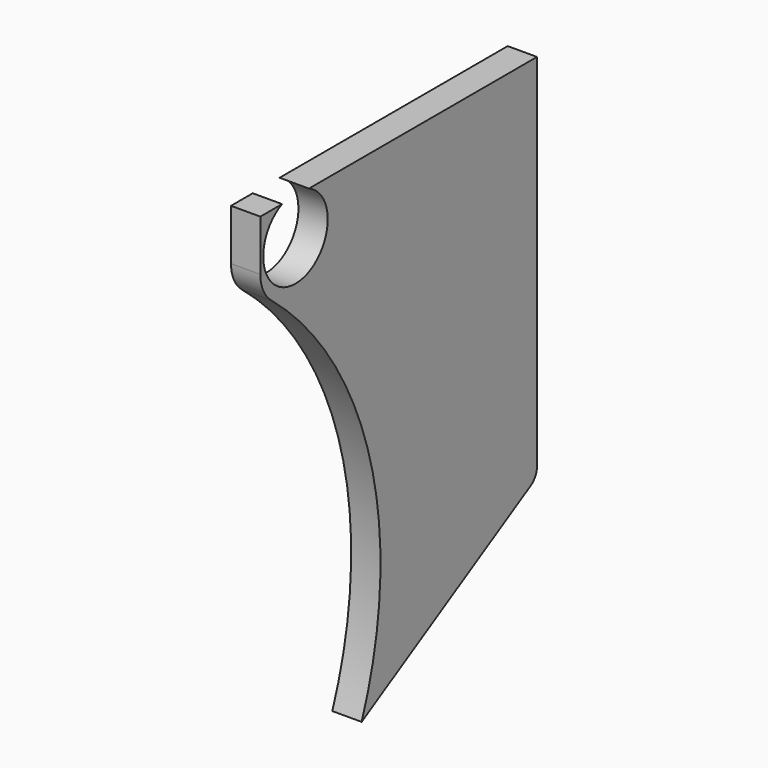
from build123d import *

# Parameters (mm, degrees)
F1_DEPTH     = 34
F2_R         = 5
F3_T         = -2.4
F5_DEPTH     = 31.6
F6_R         = 2.5
F7_DEPTH     = 34.001
F8_R         = 5
F9_T         = 2.4
F9_T3_DEPTH  = 10.7666522226
F9_T5_DEPTH  = 36.6379168457
F9_T7_DEPTH  = 39.0950180144
F9_T9_DEPTH  = 53.9897706946
F9_T11_DEPTH = 38.5655287546
F9_T13_DEPTH = 38.5655287546
F9_T15_DEPTH = 34
F9_T17_DEPTH = 38.8
F9_T20_ANGLE = 72.0602715047
F9_T22_ANGLE = 0.4928779222
F9_T24_ANGLE = 94.6188464687
F9_T26_ANGLE = 72.0602715047
F9_T28_ANGLE = 0.4928779222
F9_T30_ANGLE = 94.6188464687
F9_T32_ANGLE = 60.000000001
F9_T34_ANGLE = 60.000000001
F11_R        = 2.5
F12_DEPTH    = 4
F13_R        = 5
F13_R_2      = 2.5
F14_DEPTH    = 31.6
F15_W        = 10
F15_H        = 5
F16_DEPTH    = 34
F17_R        = 2.1082
F18_DEPTH    = 95.001
F19_W        = 189.8932904005
F19_H        = 164.366655983
F21_DEPTH    = 9.401
F23_DEPTH    = 25
F24_W        = 160.8902737498
F24_H        = 109.9677272141
F25_DEPTH    = 20.601
F20_R        = 5.5
F26_DEPTH    = 4.001
F28_DEPTH    = 4.001


# Not quite as in the source:
# - a shell that OpenCascade refuses in one call is made with other operations: the cavity is built on its own and cut out


with BuildPart() as f1:
    # F0 (on Right) → F1 (new body)
    with BuildSketch(Plane.YZ):
        with BuildLine():
            Line((28.1775091127, -64.6757430287), (50, -52.0765220406))
            Line((50, -52.0765220406), (50, 0))
            Line((50, 0), (0, 0))
            Line((0, 0), (0, -9.3767308061))
            ThreePointArc((0, -9.3767308061), (-15.3280037593, -98.3216569078), (-77.5220977637, -32.9149122293))
            Line((-77.5220977637, -32.9149122293), (-87.5160827584, -32.9149122293))
            ThreePointArc((-87.5160827584, -32.9149122293), (-82.2268855449, -79.5356128475), (-45, -108.0947501931))
            Line((-45, -108.0947501931), (-45, -140.5))
            Line((-45, -140.5), (-15, -140.5))
            Line((-15, -140.5), (-15, -108.0947501931))
            ThreePointArc((-15, -108.0947501931), (12.5445590619, -92.3079247214), (28.1775091127, -64.6757430287))
        make_face()
    extrude(amount=F1_DEPTH)

    # F2
    f2_edges = [f1.edges().sort_by_distance(p)[0] for p in [
        (17, 50, -52.076522),
        (17, 0, -9.376731),
    ]]
    fillet(f2_edges, radius=F2_R)

    # F3
    f3_openings = [f1.faces().sort_by_distance(p)[0] for p in [
        (17, 25, 0),
        (17, -16.449744, -98.64813),
        (17, 0.485259, -9.076135),
        (17, 0, -3.463693),
        (17, -82.51909, -32.914912),
        (17, -30, -140.5),
    ]]
    offset(amount=F3_T, openings=f3_openings, kind=Kind.INTERSECTION)

    # F4 (on face) → F5 (join, through all)
    with BuildSketch(Plane.YZ.offset(34)):
        with BuildLine():
            Line((-17.9050913084, -99.0302272455), (-17.9050913084, -108.768300841))
            ThreePointArc((-17.9050913084, -108.768300841), (12.6426107824, -92.2090955323), (28.8888176814, -61.493787543))
            Line((28.8888176814, -61.493787543), (17.0581943263, -68.3242011218))
            ThreePointArc((17.0581943263, -68.3242011218), (3.323976492, -87.9442036517), (-17.9050913084, -99.0302272455))
        make_face()
    extrude(amount=-F5_DEPTH)

    # F6 (on face) → F7 (cut, through all)
    with BuildSketch(Plane(origin=(0, 0, 0), x_dir=(0, -1, 0), z_dir=(-1, 0, 0))):
        with Locations((-6, -5)):
            Circle(F6_R)
        with Locations((-15.772, -82.60931)):
            Circle(F6_R)
    extrude(amount=-F7_DEPTH, mode=Mode.SUBTRACT)

    # F8
    f8_edges = [f1.edges().sort_by_distance(p)[0] for p in [
        (17, -17.905091, -99.030227),
    ]]
    fillet(f8_edges, radius=F8_R)

    # F9: shell of thickness 2.4, made by hand


with BuildPart() as f9_core1:
    # F9_t2: copy of F1
    add(f1.part)

    # the walls: a layer under each face that stays
    f9_faces = [f9_core1.faces().sort_by_distance(p)[0] for p in [
        (31.5714285714, 9.4533353128, -81.5227589639),
        (31.6, -26.6376443104, -122.5691520382),
        (17, -16.9486299393, -99.860595178),
        (28.3333333333, -85.8504185926, -32.9149122293),
        (2.4, -26.6376443104, -122.5691520382),
        (34, -20, -117.0833333333),
        (32.8, 0.4852593781, -9.0761346936),
        (31.6, 23.8, -34.1621005609),
        (0, -20, -117.0833333333),
        (17, 31.6790971631, -59.8828189331),
        (1.2, 0.4852593781, -9.0761346936),
        (2.4, 23.8, -34.1621005609),
        (17, -17.9050913084, -105.7849747297),
        (17, -17.6524314389, -108.7157351195),
        (17, -17.4, -124.5810415771),
        (31.5714285714, -42.8571428571, -140.5),
        (17, -42.6, -123.3524909928),
        (17, -79.8554185962, -78.8478289755),
        (17, -82.2268855449, -79.5356128475),
        (17, 37.8387545563, -59.0978203711),
        (17, 49.3301270189, -51.6897706946),
        (17, 50, -24.5948853473),
        (17, -15, -124.2973750966),
        (32.8666666667, 48.3333333333, 0),
        (32.8, 0, -3.4636934457),
        (17, -45, -124.2973750966),
        (17, 18.272, -82.60931),
        (32.8, 8.5, -5),
        (17, 47.6, -24.5948853473),
        (17, 47.2516660498, -50.4897706946),
        (1.2, 0, -3.4636934457),
        (1.2, 8.5, -5),
    ]]
    thicken(f9_faces, amount=-F9_T, mode=Mode.SUBTRACT)

    # F9_s4 → F9_t3 (cut)
    with BuildSketch(Plane.XY.offset(-111.168300841)):
        Polygon((31.576, -17.9290913084), (34, -17.9050913084), (34, -15.5050913084), (31.6, -15.5050913084), align=None)
        Polygon((2.424, -17.9290913084), (0, -17.9050913084), (0, -15.5050913084), (2.4, -15.5050913084), align=None)
    extrude(amount=F9_T3_DEPTH, mode=Mode.SUBTRACT)

    # F9_s6 → F9_t5 (cut)
    with BuildSketch(Plane.XY.offset(-142.9)):
        Polygon((31.576, -17.424), (34, -17.4), (34, -15), (31.6, -15), align=None)
        Polygon((2.424, -17.424), (0, -17.4), (0, -15), (2.4, -15), align=None)
    extrude(amount=F9_T5_DEPTH, mode=Mode.SUBTRACT)

    # F9_s8 → F9_t7 (cut)
    with BuildSketch(Plane.XY.offset(-142.9)):
        Polygon((31.576, -42.576), (34, -42.6), (34, -45), (31.6, -45), align=None)
        Polygon((2.424, -42.576), (0, -42.6), (0, -45), (2.4, -45), align=None)
    extrude(amount=F9_T7_DEPTH, mode=Mode.SUBTRACT)

    # F9_s10 → F9_t9 (cut)
    with BuildSketch(Plane.XY.offset(-51.5897706946)):
        Polygon((31.576, 47.576), (34, 47.6), (34, 50), (31.6, 50), align=None)
        Polygon((2.424, 47.576), (0, 47.6), (0, 50), (2.4, 50), align=None)
    extrude(amount=F9_T9_DEPTH, mode=Mode.SUBTRACT)

    # F9_s12 → F9_t11 (cut)
    with BuildSketch(Plane(origin=(0, 14.5286654552, 8.3881289115), x_dir=(1, 0, 0), z_dir=(0, -0.8660254038, -0.5))):
        Polygon((31.576, -67.6755910279), (34, -67.6995910279), (34, -70.0995910279), (31.6, -70.0995910279), align=None)
    extrude(amount=F9_T11_DEPTH, mode=Mode.SUBTRACT)

    # F9_s14 → F9_t13 (cut)
    with BuildSketch(Plane(origin=(0, -18.8700621567, -10.8946354658), x_dir=(1, 0, 0), z_dir=(0, 0.8660254038, 0.5))):
        Polygon((2.424, 67.6755910279), (2.4, 70.0995910279), (0, 70.0995910279), (0, 67.6995910279), align=None)
    extrude(amount=F9_T13_DEPTH, mode=Mode.SUBTRACT)

    # F9_s16 → F9_t15 (cut)
    with BuildSketch(Plane.YZ):
        Polygon((-17.41896, -108.6855479875), (-17.904, -106.3155998281), (-15, -105.6918510958), (-15, -108.6620831543), align=None)
    extrude(amount=F9_T15_DEPTH, mode=Mode.SUBTRACT)

    # F9_s18 → F9_t17 (cut)
    with BuildSketch(Plane.YZ.offset(-2.4)):
        Polygon((-45.03, -108.1179880932), (-44.4, -105.7709601854), (-42.6, -106.2357181869), (-42.6, -108.0947501931), align=None)
    extrude(amount=F9_T17_DEPTH, mode=Mode.SUBTRACT)

    # F9_s19 → F9_t20 (revolve, cut)
    with BuildSketch(Plane(origin=(0, -41.8058245271, -13.5349325593), x_dir=(1, 0, 0), z_dir=(0, 0.9513810562, 0.3080163728))):
        Polygon((31.576, 88.8045616247), (34, 88.8285616247), (34, 91.2285616247), (31.6, 91.2285616247), align=None)
    revolve(axis=Axis((31.6, -12.9050913084, -102.8016486184), (1, 0, 0)), revolution_arc=F9_T20_ANGLE, mode=Mode.SUBTRACT)

    # F9_s21 → F9_t22 (revolve, cut)
    with BuildSketch(Plane(origin=(0, -38.6531269844, -7.9550716089), x_dir=(1, 0, 0), z_dir=(0, -0.9794716807, -0.2015818115))):
        Polygon((31.576, -102.9501296884), (34, -102.9261296884), (34, -100.5261296884), (31.6, -100.5261296884), align=None)
    revolve(axis=Axis((31.6, -30, -50), (1, 0, 0)), revolution_arc=F9_T22_ANGLE, mode=Mode.SUBTRACT)

    # F9_s23 → F9_t24 (revolve, cut)
    with BuildSketch(Plane(origin=(0, -17.8918491238, 4.0109842757), x_dir=(1, 0, 0), z_dir=(0, 0.9757809372, -0.21875))):
        Polygon((31.576, 112.9275468625), (34, 112.9515468625), (34, 115.3515468625), (31.6, 115.3515468625), align=None)
    revolve(axis=Axis((31.6, -30, -50), (-1, 0, 0)), revolution_arc=F9_T24_ANGLE, mode=Mode.SUBTRACT)

    # F9_s25 → F9_t26 (revolve, cut)
    with BuildSketch(Plane(origin=(0, -41.8058245271, -13.5349325593), x_dir=(1, 0, 0), z_dir=(0, 0.9513810562, 0.3080163728))):
        Polygon((2.424, 88.8045616247), (2.4, 91.2285616247), (0, 91.2285616247), (0, 88.8285616247), align=None)
    revolve(axis=Axis((2.4, -12.9050913084, -102.8016486184), (1, 0, 0)), revolution_arc=F9_T26_ANGLE, mode=Mode.SUBTRACT)

    # F9_s27 → F9_t28 (revolve, cut)
    with BuildSketch(Plane(origin=(0, -38.6531269844, -7.9550716089), x_dir=(1, 0, 0), z_dir=(0, -0.9794716807, -0.2015818115))):
        Polygon((2.424, -102.9501296884), (0, -102.9261296884), (0, -100.5261296884), (2.4, -100.5261296884), align=None)
    revolve(axis=Axis((2.4, -30, -50), (1, 0, 0)), revolution_arc=F9_T28_ANGLE, mode=Mode.SUBTRACT)

    # F9_s29 → F9_t30 (revolve, cut)
    with BuildSketch(Plane(origin=(0, -17.8918491238, 4.0109842757), x_dir=(1, 0, 0), z_dir=(0, 0.9757809372, -0.21875))):
        Polygon((2.424, 112.9275468625), (0, 112.9515468625), (0, 115.3515468625), (2.4, 115.3515468625), align=None)
    revolve(axis=Axis((2.4, -30, -50), (-1, 0, 0)), revolution_arc=F9_T30_ANGLE, mode=Mode.SUBTRACT)

    # F9_s31 → F9_t32 (revolve, cut)
    with BuildSketch(Plane(origin=(0, 12.4502044861, 7.1881289115), x_dir=(1, 0, 0), z_dir=(0, -0.8660254038, -0.5))):
        Polygon((31.576, -67.6755910279), (34, -67.6995910279), (34, -70.0995910279), (31.6, -70.0995910279), align=None)
    revolve(axis=Axis((31.6, 45, -49.1897706946), (1, 0, 0)), revolution_arc=F9_T32_ANGLE, mode=Mode.SUBTRACT)

    # F9_s33 → F9_t34 (revolve, cut)
    with BuildSketch(Plane(origin=(0, 12.4502044861, 7.1881289115), x_dir=(1, 0, 0), z_dir=(0, -0.8660254038, -0.5))):
        Polygon((2.424, -67.6755910279), (0, -67.6995910279), (0, -70.0995910279), (2.4, -70.0995910279), align=None)
    revolve(axis=Axis((2.4, 45, -49.1897706946), (1, 0, 0)), revolution_arc=F9_T34_ANGLE, mode=Mode.SUBTRACT)


with BuildPart() as f1_1:
    add(f1.part)

    # what is left inside the walls is the cavity
    f9_cavity = [f9_core1.part.solids().sort_by_distance(p)[0] for p in [
        (21.866667, 25.090457, -73.709958),
        (21.866667, 2.64665, -100.312194),
    ]]
    add(f9_cavity, mode=Mode.SUBTRACT)

    # F11 (on offset) → F12 (join)
    with BuildSketch(Plane.YZ.offset(9.4)):
        with BuildLine():
            Line((47.6, -49.1897706946), (47.6, 0))
            Line((47.6, 0), (0, 0))
            Line((0, 0), (0, -6.9273868914))
            ThreePointArc((0, -6.9273868914), (0.4852593781, -9.0761346936), (1.8468468468, -10.8078024868))
            ThreePointArc((1.8468468468, -10.8078024868), (18.82146463, -37.0881995298), (17.0581943263, -68.3242011218))
            Line((17.0581943263, -68.3242011218), (46.3, -51.4414367444))
            ThreePointArc((46.3, -51.4414367444), (47.2516660498, -50.4897706946), (47.6, -49.1897706946))
        make_face()
        with Locations((6, -5)):
            Circle(F11_R, mode=Mode.SUBTRACT)
    extrude(amount=F12_DEPTH)

    # F13 (on face) → F14 (join, through all)
    with BuildSketch(Plane(origin=(0, 0, 0), x_dir=(0, -1, 0), z_dir=(-1, 0, 0))):
        with Locations((-6, -5)):
            Circle(F13_R)
        with Locations((-6, -5)):
            Circle(F13_R_2, mode=Mode.SUBTRACT)
    extrude(amount=-F14_DEPTH)

    # F15 (on face) → F16 (join, through all)
    with BuildSketch(Plane(origin=(0, 0, 0), x_dir=(0, -1, 0), z_dir=(-1, 0, 0))):
        with Locations((50, -111.9852015376)):
            Rectangle(F15_W, F15_H)
        with Locations((10, -111.9852015376)):
            Rectangle(F15_W, F15_H)
    extrude(amount=-F16_DEPTH)

    # F17 (on face) → F18 (cut, through all)
    with BuildSketch(Plane.XZ.offset(45)):
        with Locations((17, -127.4926007688)):
            Circle(F17_R)
    extrude(amount=-F18_DEPTH, mode=Mode.SUBTRACT)

    # F19 (on face) → F21 (cut, through all)
    with BuildSketch(Plane(origin=(9.4, 0, 0), x_dir=(0, -1, 0), z_dir=(-1, 0, 0))):
        with Locations((31.2468931079, -71.6645303182)):
            Rectangle(F19_W, F19_H)
    extrude(amount=F21_DEPTH, mode=Mode.SUBTRACT)

    # F22 (on face) → F23 (cut)
    with BuildSketch(Plane(origin=(9.4, 0, 0), x_dir=(0, -1, 0), z_dir=(-1, 0, 0))):
        with BuildLine():
            Line((-17.0581943263, -68.3242011218), (-46.3, -51.4414367444))
            ThreePointArc((-46.3, -51.4414367444), (-47.2516660498, -50.4897706946), (-47.6, -49.1897706946))
            Line((-47.6, -49.1897706946), (-47.6, 0))
            Line((-47.6, 0), (-64.246557653, 0))
            Line((-64.246557653, 0), (-89.291639626, -69.9864493248))
            Line((-89.291639626, -69.9864493248), (20.7843445241, -157.047316432))
            Line((20.7843445241, -157.047316432), (124.3782043457, -131.2076151371))
            Line((124.3782043457, -131.2076151371), (97.628891468, -13.250593096))
            Line((97.628891468, -13.250593096), (-17.0581943263, -68.3242011218))
        make_face()
    extrude(amount=-F23_DEPTH, mode=Mode.SUBTRACT)

    # F24 (on face) → F25 (cut, through all)
    with BuildSketch(Plane.YZ.offset(13.4)):
        with Locations((17.4953527749, -42.2205235809)):
            Rectangle(F24_W, F24_H)
    extrude(amount=F25_DEPTH, mode=Mode.SUBTRACT)

    # F20 (on face) → F26 (cut, through all)
    with BuildSketch(Plane(origin=(9.4, 0, 0), x_dir=(0, -1, 0), z_dir=(-1, 0, 0))):
        with Locations((-6, -5)):
            Circle(F20_R)
    extrude(amount=-F26_DEPTH, mode=Mode.SUBTRACT)

    # F27 (on face) → F28 (cut, through all)
    with BuildSketch(Plane(origin=(9.4, 0, 0), x_dir=(0, -1, 0), z_dir=(-1, 0, 0))):
        with BuildLine():
            ThreePointArc((-46.1, -51.0950265829), (-46.9052558883, -50.2897706946), (-47.2, -49.1897706946))
            Line((-47.2, -49.1897706946), (-47.2, 2.7465141902))
            Line((-47.2, 2.7465141902), (-59.5964565873, 2.7465141902))
            Line((-59.5964565873, 2.7465141902), (-59.5964565873, -69.7395056486))
            Line((-59.5964565873, -69.7395056486), (-14.8213052426, -70.3015608949))
            Line((-14.8213052426, -70.3015608949), (-14.8213052426, -69.153789421))
            Line((-14.8213052426, -69.153789421), (-46.1, -51.0950265829))
        make_face()
    extrude(amount=-F28_DEPTH, mode=Mode.SUBTRACT)


solid = f1_1.part
